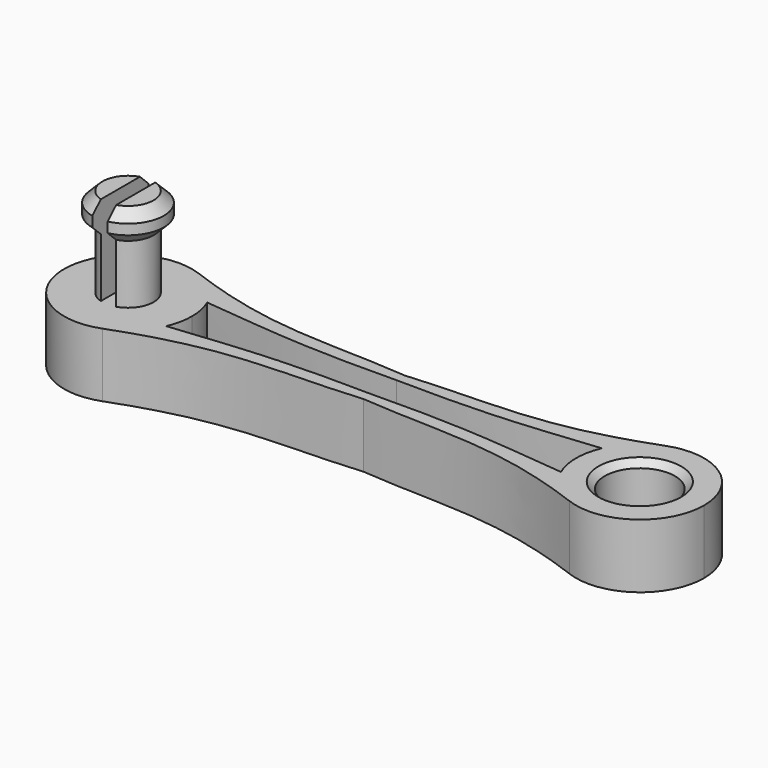
from build123d import *

# Parameters (mm, degrees)
F2_DEPTH = 6.35
F1_W     = 1.778
F1_H     = 3.048
F1_H_2   = 5.842
F1_W_2   = 0.762
F5_DEPTH = 12.7
F6_DEPTH = 2.54


# Not quite as in the source:
# - a feature names something its author has since deleted; it is built from what else it names


with BuildPart() as f2:
    # F0 (on Top) → F2 (new body)
    with BuildSketch(Plane.XY):
        with BuildLine():
            ThreePointArc((-19.5801208863, -2.5399817128), (-19.1839428746, -1.2973564714), (-19.05, 0))
            ThreePointArc((-19.05, 0), (-19.1839428746, 1.2973564714), (-19.5801208863, 2.5399817128))
            ThreePointArc((-19.5801208863, 2.5399817128), (-21.0323461368, 4.6093491657), (-23.1768579109, 5.9481206487))
            ThreePointArc((-23.1768579109, 5.9481206487), (-31.75, 0), (-23.1768579109, -5.9481206487))
            ThreePointArc((-23.1768579109, -5.9481206487), (-21.0323461368, -4.6093491657), (-19.5801208863, -2.5399817128))
        make_face()
        with BuildLine():
            ThreePointArc((-23.1768579109, 5.9481206487), (-21.0323461368, 4.6093491657), (-19.5801208863, 2.5399817128))
            add(Edge.make_bspline(
                [(0, 1.524), (-9.0764431036, 1.3546369813), (-12.8672626316, 1.8652065321), (-19.5801208863, 2.5399817128)],
                knots=[0, 0, 0, 0, 19.6064620154, 19.6064620154, 19.6064620154, 19.6064620154], degree=3))
            add(Edge.make_bspline(
                [(0, 1.524), (9.0764431036, 1.3546369813), (12.8672626316, 1.8652065321), (19.5801208863, 2.5399817128)],
                knots=[0, 0, 0, 0, 19.6064620154, 19.6064620154, 19.6064620154, 19.6064620154], degree=3))
            ThreePointArc((19.5801208863, 2.5399817128), (21.0323461368, 4.6093491657), (23.1768579109, 5.9481206487))
            add(Edge.make_bspline(
                [(0, 2.54), (8.1250406802, 3.246476237), (13.1090918084, 2.1852389104), (23.1768579109, 5.9481206487)],
                knots=[0, 0, 0, 0, 23.4260971776, 23.4260971776, 23.4260971776, 23.4260971776], degree=3))
            add(Edge.make_bspline(
                [(0, 2.54), (-8.1250406802, 3.246476237), (-13.1090918084, 2.1852389104), (-23.1768579109, 5.9481206487)],
                knots=[0, 0, 0, 0, 23.4260971776, 23.4260971776, 23.4260971776, 23.4260971776], degree=3))
        make_face()
        with BuildLine():
            add(Edge.make_bspline(
                [(0, -1.524), (-9.0764431036, -1.3546369813), (-12.8672626316, -1.8652065321), (-19.5801208863, -2.5399817128)],
                knots=[0, 0, 0, 0, 19.6064620154, 19.6064620154, 19.6064620154, 19.6064620154], degree=3))
            ThreePointArc((-19.5801208863, -2.5399817128), (-21.0323461368, -4.6093491657), (-23.1768579109, -5.9481206487))
            add(Edge.make_bspline(
                [(0, -2.54), (-8.1250406802, -3.246476237), (-13.1090918084, -2.1852389104), (-23.1768579109, -5.9481206487)],
                knots=[0, 0, 0, 0, 23.4260971776, 23.4260971776, 23.4260971776, 23.4260971776], degree=3))
            add(Edge.make_bspline(
                [(0, -2.54), (8.1250406802, -3.246476237), (13.1090918084, -2.1852389104), (23.1768579109, -5.9481206487)],
                knots=[0, 0, 0, 0, 23.4260971776, 23.4260971776, 23.4260971776, 23.4260971776], degree=3))
            ThreePointArc((23.1768579109, -5.9481206487), (21.0323461368, -4.6093491657), (19.5801208863, -2.5399817128))
            add(Edge.make_bspline(
                [(0, -1.524), (9.0764431036, -1.3546369813), (12.8672626316, -1.8652065321), (19.5801208863, -2.5399817128)],
                knots=[0, 0, 0, 0, 19.6064620154, 19.6064620154, 19.6064620154, 19.6064620154], degree=3))
        make_face()
        with BuildLine():
            ThreePointArc((23.1768579109, 5.9481206487), (21.0323461368, 4.6093491657), (19.5801208863, 2.5399817128))
            ThreePointArc((19.5801208863, 2.5399817128), (19.05, 0), (19.5801208863, -2.5399817128))
            ThreePointArc((19.5801208863, -2.5399817128), (21.0323461368, -4.6093491657), (23.1768579109, -5.9481206487))
            ThreePointArc((23.1768579109, -5.9481206487), (29.019775389, -5.2172527381), (31.75, 0))
            ThreePointArc((31.75, 0), (29.019775389, 5.2172527381), (23.1768579109, 5.9481206487))
        make_face()
    extrude(amount=F2_DEPTH)

    # F1 (on Front) → F3 (revolve, cut)
    with BuildSketch(Plane.XZ):
        Polygon((25.376161883, 6.35), (25.376161883, 0), (29.490961883, 0), (28.855961883, 0.635), (28.855961883, 5.715), (29.490961883, 6.35), align=None)
    revolve(axis=Axis((25.376161883, 0, 3.175), (0, 0, 1)), mode=Mode.SUBTRACT)

    # F1 (on Front) → F4 (revolve)
    with BuildSketch(Plane.XZ):
        Polygon((-22.86, 15.24), (-22.86, 12.192), (-21.844, 13.208), (-21.844, 14.224), align=None)
        with Locations((-23.749, 13.716)):
            Rectangle(F1_W, F1_H)
        with Locations((-27.051, 13.716)):
            Rectangle(F1_W, F1_H)
        Polygon((-28.956, 13.208), (-27.94, 12.192), (-27.94, 15.24), (-28.956, 14.224), align=None)
        with Locations((-27.051, 9.271)):
            Rectangle(F1_W, F1_H_2)
        with Locations((-23.749, 9.271)):
            Rectangle(F1_W, F1_H_2)
    revolve(axis=Axis((-25.4, 0, 10.795), (0, 0, 1)))

    # F1 (on Front) → F5 (cut, symmetric)
    with BuildSketch(Plane.XZ):
        with Locations((-25.019, 13.716)):
            Rectangle(F1_W_2, F1_H)
        with Locations((-25.781, 13.716)):
            Rectangle(F1_W_2, F1_H)
        with Locations((-25.019, 9.271)):
            Rectangle(F1_W_2, F1_H_2)
        with Locations((-25.781, 9.271)):
            Rectangle(F1_W_2, F1_H_2)
    extrude(amount=F5_DEPTH, both=True, mode=Mode.SUBTRACT)

    # F0 (on Top) → F6 (join)
    with BuildSketch(Plane.XY):
        with BuildLine():
            ThreePointArc((-19.5801208863, 2.5399817128), (-19.1839428746, 1.2973564714), (-19.05, 0))
            ThreePointArc((-19.05, 0), (-19.1839428746, -1.2973564714), (-19.5801208863, -2.5399817128))
            add(Edge.make_bspline(
                [(0, -1.524), (-9.0764431036, -1.3546369813), (-12.8672626316, -1.8652065321), (-19.5801208863, -2.5399817128)],
                knots=[0, 0, 0, 0, 19.6064620154, 19.6064620154, 19.6064620154, 19.6064620154], degree=3))
            add(Edge.make_bspline(
                [(0, -1.524), (9.0764431036, -1.3546369813), (12.8672626316, -1.8652065321), (19.5801208863, -2.5399817128)],
                knots=[0, 0, 0, 0, 19.6064620154, 19.6064620154, 19.6064620154, 19.6064620154], degree=3))
            ThreePointArc((19.5801208863, -2.5399817128), (19.05, 0), (19.5801208863, 2.5399817128))
            add(Edge.make_bspline(
                [(0, 1.524), (9.0764431036, 1.3546369813), (12.8672626316, 1.8652065321), (19.5801208863, 2.5399817128)],
                knots=[0, 0, 0, 0, 19.6064620154, 19.6064620154, 19.6064620154, 19.6064620154], degree=3))
            add(Edge.make_bspline(
                [(0, 1.524), (-9.0764431036, 1.3546369813), (-12.8672626316, 1.8652065321), (-19.5801208863, 2.5399817128)],
                knots=[0, 0, 0, 0, 19.6064620154, 19.6064620154, 19.6064620154, 19.6064620154], degree=3))
        make_face()
    extrude(amount=F6_DEPTH)


solid = f2.part
